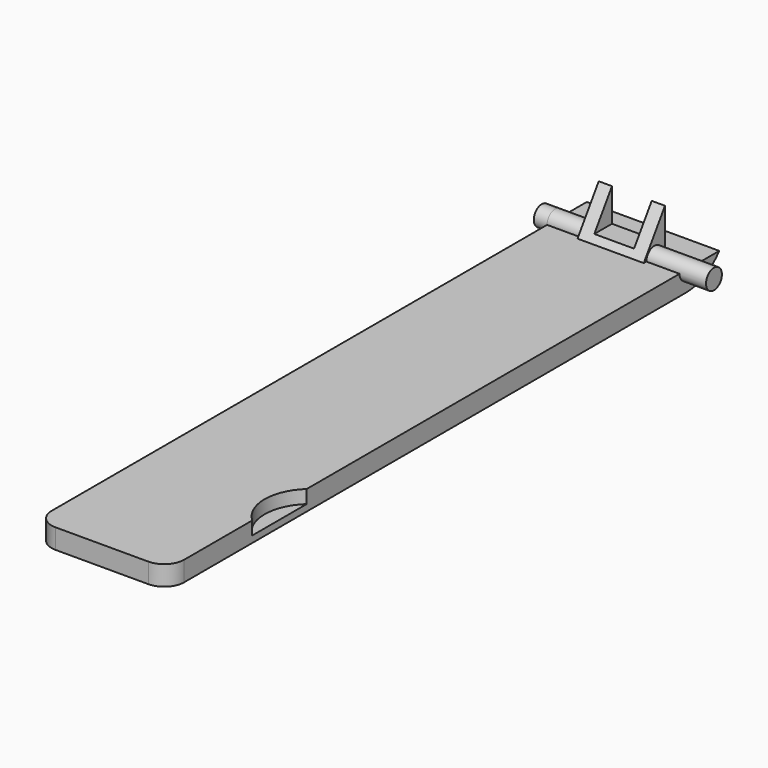
from build123d import *

# Parameters (mm, degrees)
F0_W         = 10
F0_H         = 52
F1_DEPTH     = 1.5
F2_W         = 5
F2_H         = 2
F3_DEPTH     = 3
F5_DEPTH     = 6
F7_DEPTH     = 1
F8_DEPTH     = 12
F9_R         = 1.5
F10_R        = 1.5
F12_DEPTH    = 1
F13_T1_DEPTH = 25.612494996
F14_W        = 3
F14_H        = 2.5
F15_DEPTH    = 5


# Not quite as in the source:
# - a fillet or chamfer that OpenCascade refuses, or shapes differently, is made with other operations: its cross-section is extruded or revolved along the edge and cut away or added


with BuildPart() as f1:
    # F0 (on Top) → F1 (new body)
    with BuildSketch(Plane.XY):
        with Locations((-5, 26)):
            Rectangle(F0_W, F0_H)
    extrude(amount=F1_DEPTH)

    # F2 (on face) → F3 (join)
    with BuildSketch(Plane.XY.offset(1.5)):
        with Locations((-5, 49)):
            Rectangle(F2_W, F2_H)
    extrude(amount=F3_DEPTH)

    # F4 (on face) → F5 (cut)
    with BuildSketch(Plane(origin=(-7.5, 0, 0), x_dir=(0, -1, 0), z_dir=(-1, 0, 0))):
        Polygon((-48, 4.5), (-50, 4.5), (-48, 1.5), align=None)
    extrude(amount=-F5_DEPTH, mode=Mode.SUBTRACT)

    # F6 (on face) → F7 (join)
    with BuildSketch(Plane(origin=(-10, 0, 0), x_dir=(0, -1, 0), z_dir=(-1, 0, 0))):
        with BuildLine():
            Line((-49.75, 1.5), (-48.25, 1.5))
            ThreePointArc((-48.25, 1.5), (-49, 2.25), (-49.75, 1.5))
        make_face()
        with BuildLine():
            ThreePointArc((-49.75, 1.5), (-49, 0.75), (-48.25, 1.5))
            Line((-48.25, 1.5), (-49.75, 1.5))
        make_face()
    extrude(amount=F7_DEPTH)

    # F6 (on face) → F8 (join)
    with BuildSketch(Plane(origin=(-10, 0, 0), x_dir=(0, -1, 0), z_dir=(-1, 0, 0))):
        with BuildLine():
            Line((-49.75, 1.5), (-48.25, 1.5))
            ThreePointArc((-48.25, 1.5), (-49, 2.25), (-49.75, 1.5))
        make_face()
        with BuildLine():
            ThreePointArc((-49.75, 1.5), (-49, 0.75), (-48.25, 1.5))
            Line((-48.25, 1.5), (-49.75, 1.5))
        make_face()
    extrude(amount=-F8_DEPTH)

    # F9
    f9_edges = [f1.edges().sort_by_distance(p)[0] for p in [
        (-10, 0, 0.75),
    ]]
    fillet(f9_edges, radius=F9_R)

    # F10
    f10_edges = [f1.edges().sort_by_distance(p)[0] for p in [
        (0, 0, 0.75),
    ]]
    fillet(f10_edges, radius=F10_R)

    # F11 (on face) → F12 (cut)
    with BuildSketch(Plane.XY.offset(1.5)):
        with BuildLine():
            Line((0, 7.928885867), (0, 13.071114133))
            ThreePointArc((0, 13.071114133), (-1.1252637799, 10.5), (0, 7.928885867))
        make_face()
    extrude(amount=-F12_DEPTH, mode=Mode.SUBTRACT)

    # F13: fillet of radius 4 on 1 edges, made by hand

    # F13_s2 → F13_t1 (cut)
    with BuildSketch(Plane.YZ.offset(-17.806247498)):
        with BuildLine():
            ThreePointArc((48.8775010008, 0), (50.6095518084, 0.3944487245), (52, 1.5))
            Line((52, 1.5), (52, 0))
            Line((52, 0), (48.8775010008, 0))
        make_face()
    extrude(amount=F13_T1_DEPTH, mode=Mode.SUBTRACT)

    # F14 (on face) → F15 (cut)
    with BuildSketch(Plane(origin=(0, 50, 0), x_dir=(-1, 0, 0), z_dir=(0, 1, 0))):
        with Locations((5, 3.25)):
            Rectangle(F14_W, F14_H)
    extrude(amount=-F15_DEPTH, mode=Mode.SUBTRACT)


solid = f1.part
